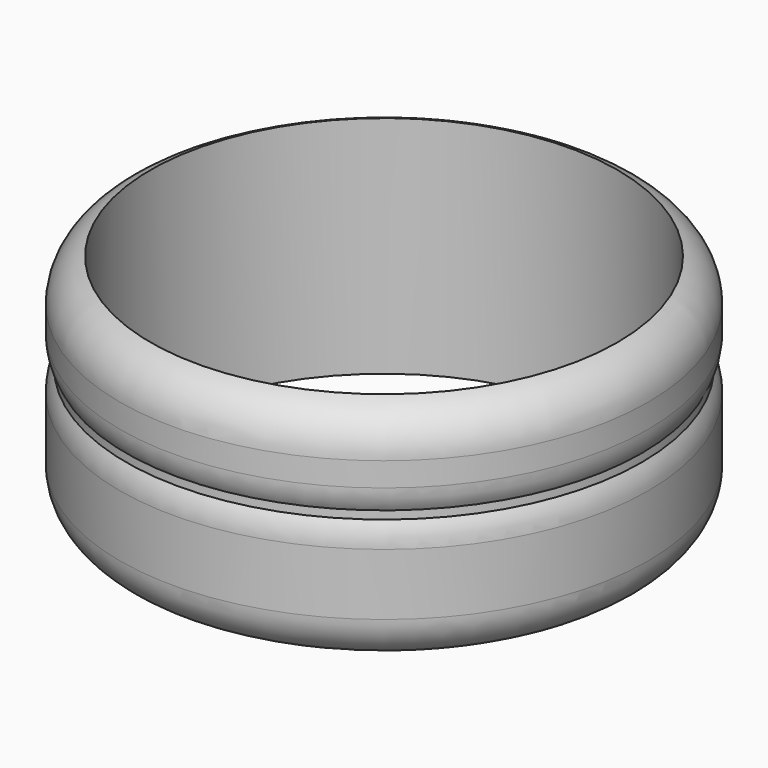
from build123d import *

# Parameters (mm, degrees)
F0_R     = 29.8077198066
F1_DEPTH = 25.4
F2_R     = 26.3502536292
F3_DEPTH = 25.4
F4_W     = 2.8885006905
F4_H     = 0.9121578187


# Not quite as in the source:
# - a fillet or chamfer that OpenCascade refuses, or shapes differently, is made with other operations: its cross-section is extruded or revolved along the edge and cut away or added


with BuildPart() as f1:
    # F0 (on Top) → F1 (new body)
    with BuildSketch(Plane.XY):
        Circle(F0_R)
    extrude(amount=F1_DEPTH)

    # F2 (on face) → F3 (cut)
    with BuildSketch(Plane.XY.offset(25.4)):
        Circle(F2_R)
    extrude(amount=-F3_DEPTH, mode=Mode.SUBTRACT)

    # F4 (on Right) → F6 (revolve, cut)
    with BuildSketch(Plane.YZ):
        with Locations((-30.5377691984, 14.828927815)):
            Rectangle(F4_W, F4_H)
    revolve(axis=Axis((0, 0, 31.8907126784), (0, 0, 1)), mode=Mode.SUBTRACT)

    # F7: fillet of radius 5.08 on 6 edges, made by hand

    # F7_s1 → F7_t2 (revolve, cut)
    with BuildSketch(Plane.XZ):
        with BuildLine():
            ThreePointArc((29.0935188532, 15.2850067243), (29.6259163705, 16.5354769537), (29.8077198066, 17.8823512692))
            Line((29.8077198066, 17.8823512692), (29.9093198066, 17.8823512692))
            Line((29.9093198066, 17.8823512692), (29.9093198066, 15.2850067243))
            Line((29.9093198066, 15.2850067243), (29.8077198066, 15.1834067243))
            ThreePointArc((29.8077198066, 15.1834067243), (29.4506193299, 15.1834067243), (29.1808348341, 15.2330598334))
            Line((29.1808348341, 15.2330598334), (29.0935188532, 15.2850067243))
        make_face()
    revolve(axis=Axis((0, 0, 15.2850067243), (0, 0, -1)), mode=Mode.SUBTRACT)

    # F7_s3 → F7_t4 (revolve, cut)
    with BuildSketch(Plane.XZ):
        with BuildLine():
            ThreePointArc((26.3502536292, 25.4), (28.8537876574, 23.5495222224), (29.8077198066, 20.5860843387))
            Line((29.8077198066, 20.5860843387), (29.9093198066, 20.5860843387))
            Line((29.9093198066, 20.5860843387), (29.9093198066, 25.4))
            Line((29.9093198066, 25.4), (29.8077198066, 25.5016))
            ThreePointArc((29.8077198066, 25.5016), (28.0789867179, 25.5016), (26.3827043057, 25.4962783132))
            Line((26.3827043057, 25.4962783132), (26.3502536292, 25.4))
        make_face()
    revolve(axis=Axis((0, 0, 25.4), (0, 0, 1)), mode=Mode.SUBTRACT)

    # F7_s5 → F7_t6 (revolve, cut)
    with BuildSketch(Plane.XZ):
        with BuildLine():
            ThreePointArc((29.8077198066, 4.8139156613), (28.8537876574, 1.8504777776), (26.3502536292, 0))
            Line((26.3502536292, 0), (26.3827043057, -0.0962783132))
            ThreePointArc((26.3827043057, -0.0962783132), (28.0789867179, -0.1016), (29.8077198066, -0.1016))
            Line((29.8077198066, -0.1016), (29.9093198066, 0))
            Line((29.9093198066, 0), (29.9093198066, 4.8139156613))
            Line((29.9093198066, 4.8139156613), (29.8077198066, 4.8139156613))
        make_face()
    revolve(axis=Axis((0, 0, 0), (0, 0, 1)), mode=Mode.SUBTRACT)

    # F7_s7 → F7_t8 (revolve, cut)
    with BuildSketch(Plane.XZ):
        with BuildLine():
            ThreePointArc((29.8077198066, 11.7755043607), (29.6259163705, 13.1223786762), (29.0935188532, 14.3728489056))
            Line((29.0935188532, 14.3728489056), (29.1808348341, 14.4247957965))
            ThreePointArc((29.1808348341, 14.4247957965), (29.4506193299, 14.4744489056), (29.8077198066, 14.4744489056))
            Line((29.8077198066, 14.4744489056), (29.9093198066, 14.3728489056))
            Line((29.9093198066, 14.3728489056), (29.9093198066, 11.7755043607))
            Line((29.9093198066, 11.7755043607), (29.8077198066, 11.7755043607))
        make_face()
    revolve(axis=Axis((0, 0, 14.3728489056), (0, 0, -1)), mode=Mode.SUBTRACT)


solid = f1.part
